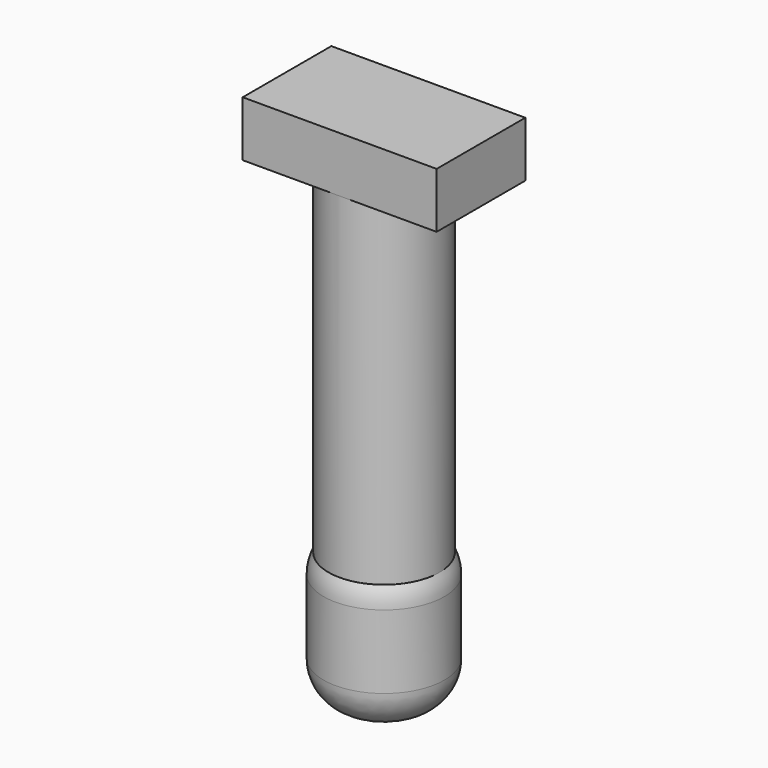
from build123d import *

# Parameters (mm, degrees)
F0_R     = 2.0955
F1_DEPTH = 12.7
F2_W     = 7.33298
F2_H     = 4.1894274764
F3_DEPTH = 2.0955
F4_R     = 2.284478014
F4_R_2   = 2.0955
F5_DEPTH = 5.08


# Not quite as in the source:
# - a fillet or chamfer that OpenCascade refuses, or shapes differently, is made with other operations: its cross-section is extruded or revolved along the edge and cut away or added


with BuildPart() as f1:
    # F0 (on Top) → F1 (new body)
    with BuildSketch(Plane.XY):
        Circle(F0_R)
    extrude(amount=F1_DEPTH)

    # F2 (on face) → F3 (join)
    with BuildSketch(Plane.XY.offset(12.7)):
        Rectangle(F2_W, F2_H)
    extrude(amount=F3_DEPTH)

    # F4 (on face) → F5 (join)
    with BuildSketch(Plane(origin=(0, 0, 0), x_dir=(1, 0, 0), z_dir=(0, 0, -1))):
        Circle(F4_R)
        Circle(F4_R_2, mode=Mode.SUBTRACT)
        Circle(F4_R_2)
    extrude(amount=F5_DEPTH)

    # F6: fillet of radius 1.5570711792 on 2 edges, made by hand

    # F6_s1 → F6_t2 (revolve, cut)
    with BuildSketch(Plane.XZ):
        with BuildLine():
            ThreePointArc((2.284478014, -0.7434996627), (2.2364941575, -0.3599294481), (2.0955, 0))
            Line((2.0955, 0), (2.284478014, 0))
            Line((2.284478014, 0), (2.284478014, -0.7434996627))
        make_face()
    revolve(axis=Axis((0, 0, 0), (0, 0, -1)), mode=Mode.SUBTRACT)

    # F6_s3 → F6_t4 (revolve, cut)
    with BuildSketch(Plane.XZ):
        with BuildLine():
            ThreePointArc((2.284478014, -3.5229288208), (1.8284224244, -4.6239444104), (0.7274068348, -5.08))
            Line((0.7274068348, -5.08), (2.284478014, -5.08))
            Line((2.284478014, -5.08), (2.284478014, -3.5229288208))
        make_face()
    revolve(axis=Axis((0, 0, -5.08), (0, 0, -1)), mode=Mode.SUBTRACT)


solid = f1.part
